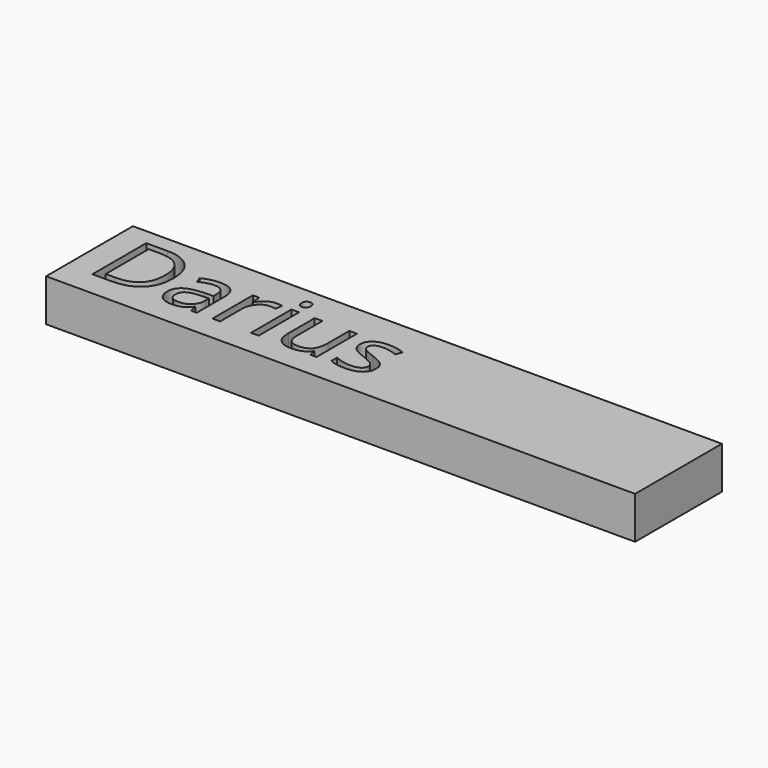
from build123d import *

# Parameters (mm, degrees)
F0_W         = 708.0286890268
F0_H         = 130.4397284985
F1_DEPTH     = 50.8
F2_TEXT_SIZE = 113.3856880996
F3_DEPTH     = 25.4


# Not quite as in the source:
# - Text() gives the source's letters only with a copy of the font that has no kerning and outlines rounded to 1/6400 em; it was checked with that copy


with BuildPart() as f1:
    # F0 (on Top) → F1 (new body)
    with BuildSketch(Plane.XY):
        with Locations((226.4820858836, -285.2579206228)):
            Rectangle(F0_W, F0_H)
    extrude(amount=-F1_DEPTH)

    # F2 (on Top) → F3 (cut)
    with BuildSketch(Plane.XY):
        with Locations((-107.2866097093, -320.0770020485)):
            Text('Darius', F2_TEXT_SIZE, font='Open Sans', text_align=(TextAlign.LEFT, TextAlign.BOTTOM))
    extrude(amount=-F3_DEPTH, mode=Mode.SUBTRACT)


solid = f1.part
